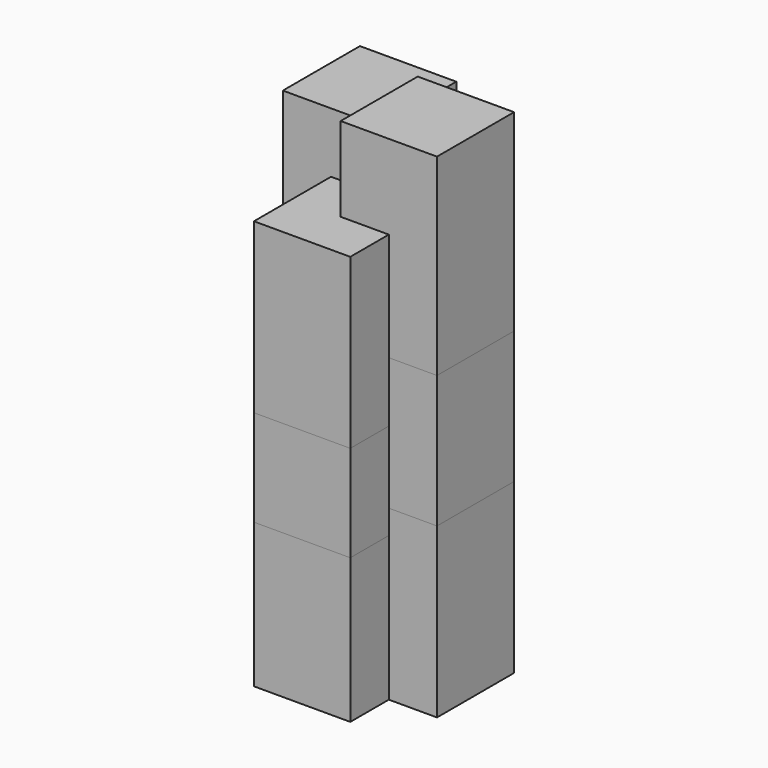
from build123d import *

# Parameters (mm, degrees)
F0_W      = 40
F0_H      = 40
F1_DEPTH  = 50
F2_W      = 40
F2_H      = 40
F3_DEPTH  = 60
F4_W      = 40
F4_H      = 40
F5_DEPTH  = 70
F7_DEPTH  = 65
F9_DEPTH  = 40
F10_W     = 40
F10_H     = 40
F11_DEPTH = 55
F14_DEPTH = 70
F16_DEPTH = 80
F17_W     = 40
F17_H     = 40
F18_DEPTH = 80


with BuildPart() as f1:
    # F0 (on Top) → F1 (new body)
    with BuildSketch(Plane.XY):
        with Locations((-20, 20)):
            Rectangle(F0_W, F0_H)
    extrude(amount=F1_DEPTH)

    # F2 (on Top) → F3 (join)
    with BuildSketch(Plane.XY):
        with Locations((0, -20)):
            Rectangle(F2_W, F2_H)
    extrude(amount=F3_DEPTH)

    # F4 (on Top) → F5 (join)
    with BuildSketch(Plane.XY):
        with Locations((20, 0)):
            Rectangle(F4_W, F4_H)
    extrude(amount=F5_DEPTH)


with BuildPart() as f7:
    # F6 (on face) → F7 (new body)
    with BuildSketch(Plane.XY.offset(50)):
        Polygon((-20, 0), (0, 0), (0, 20), (0, 40), (-40, 40), (-40, 0), align=None)
    extrude(amount=F7_DEPTH)

    # F8 (on face) → F9 (join)
    with BuildSketch(Plane.XY.offset(60)):
        Polygon((20, -40), (20, -20), (0, -20), (0, 0), (-20, 0), (-20, -40), align=None)
    extrude(amount=F9_DEPTH)

    # F10 (on face) → F11 (join)
    with BuildSketch(Plane.XY.offset(70)):
        with Locations((20, 0)):
            Rectangle(F10_W, F10_H)
    extrude(amount=F11_DEPTH)

    # F12: union 


with BuildPart() as f14:
    # F13 (on face) → F14 (new body)
    with BuildSketch(Plane.XY.offset(100)):
        Polygon((-20, -40), (20, -40), (20, -20), (0, -20), (0, 0), (-20, 0), align=None)
    extrude(amount=F14_DEPTH)

    # F15 (on face) → F16 (join)
    with BuildSketch(Plane.XY.offset(115)):
        Polygon((-40, 40), (-40, 0), (0, 0), (0, 20), (0, 40), align=None)
    extrude(amount=F16_DEPTH)

    # F17 (on face) → F18 (join)
    with BuildSketch(Plane.XY.offset(125)):
        with Locations((20, 0)):
            Rectangle(F17_W, F17_H)
    extrude(amount=F18_DEPTH)


solid = Compound([f1.part, f7.part, f14.part])
